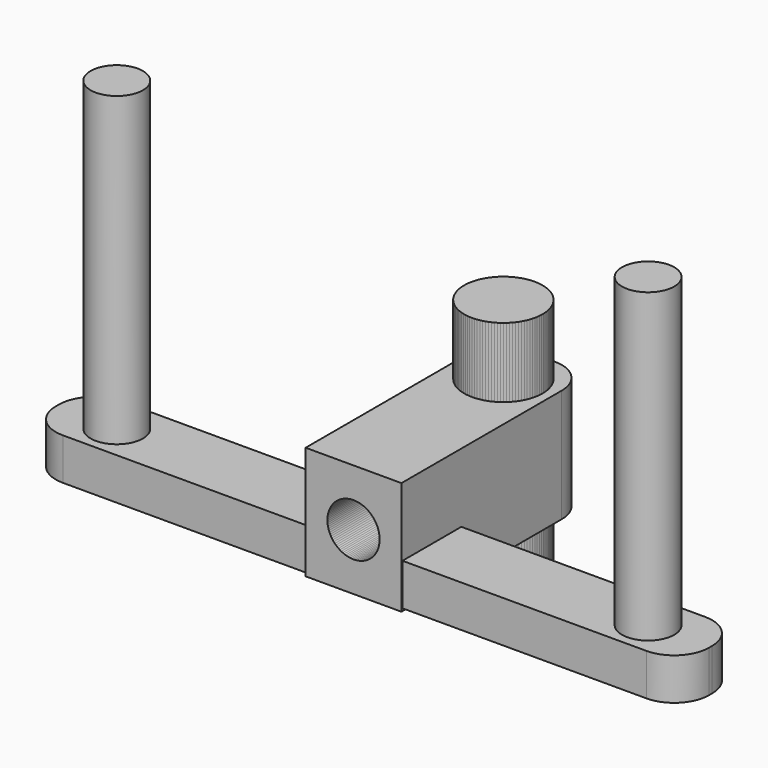
from build123d import *

# Parameters (mm, degrees)
F0_R        = 2.25
F1_DEPTH    = 4
F2_W        = 5.5
F2_H        = 5.5
F3_DEPTH    = 6.5
F4_R        = 2.25
F5_DEPTH    = 4
F6_DEPTH    = 8
F7_R        = 1.5
F8_DEPTH    = 13.5
F9_T1_DEPTH = 16.5
F11_W       = 4.2225685902
F11_H       = 2.4003293365
F12_DEPTH   = 16
F13_R       = 2
F14_R       = 1.5
F15_DEPTH   = 20


# Not quite as in the source:
# - a fillet or chamfer that OpenCascade refuses, or shapes differently, is made with other operations: its cross-section is extruded or revolved along the edge and cut away or added


with BuildPart() as f1:
    # F0 (on Top) → F1 (new body)
    with BuildSketch(Plane.XY):
        Circle(F0_R)
    extrude(amount=F1_DEPTH)

    # F2 (on face) → F3 (join)
    with BuildSketch(Plane.XY.offset(4)):
        Rectangle(F2_W, F2_H)
    extrude(amount=F3_DEPTH)

    # F4 (on face) → F5 (join)
    with BuildSketch(Plane.XY.offset(10.5)):
        Circle(F4_R)
    extrude(amount=F5_DEPTH)

    # F6 (add): a face of the model
    f6_faces = [f1.faces().sort_by_distance(p)[0] for p in [
        (0, -2.75, 7.25),
    ]]
    extrude(f6_faces, amount=F6_DEPTH)

    # F7 (on face) → F8 (cut, through all)
    with BuildSketch(Plane.XZ.offset(10.75)):
        with Locations((0, 7.25)):
            Circle(F7_R)
    extrude(amount=-F8_DEPTH, mode=Mode.SUBTRACT)

    # F9: fillet of radius 2 on 2 edges, made by hand

    # F9_s2 → F9_t1 (cut)
    with BuildSketch(Plane.XY.offset(-1)):
        with BuildLine():
            ThreePointArc((-0.75, 2.75), (-2.1642135624, 2.1642135624), (-2.75, 0.75))
            Line((-2.75, 0.75), (-2.75, 2.75))
            Line((-2.75, 2.75), (-0.75, 2.75))
        make_face()
        with BuildLine():
            ThreePointArc((0.75, 2.75), (2.1642135624, 2.1642135624), (2.75, 0.75))
            Line((2.75, 0.75), (2.75, 2.75))
            Line((2.75, 2.75), (0.75, 2.75))
        make_face()
    extrude(amount=F9_T1_DEPTH, mode=Mode.SUBTRACT)

    # F11 (on face) → F12 (join)
    with BuildSketch(Plane.YZ.offset(2.75)):
        with Locations((-8.5641460028, 5.3448951803)):
            Rectangle(F11_W, F11_H)
    extrude(amount=F12_DEPTH)

    # F13
    f13_edges = [f1.edges().sort_by_distance(p)[0] for p in [
        (18.75, -10.67543, 5.344895),
        (18.75, -6.452862, 5.344895),
    ]]
    fillet(f13_edges, radius=F13_R)

    # F14 (on face) → F15 (join)
    with BuildSketch(Plane(origin=(0, 0, 4.1447305121), x_dir=(1, 0, 0), z_dir=(0, 0, -1))):
        with Locations((15.25, 8.6754302979)):
            Circle(F14_R)
    extrude(amount=-F15_DEPTH)


with BuildPart() as f16_1:
    # F16: instance of F1
    add(f1.part.mirror(Plane.YZ))


solid = Compound([f1.part, f16_1.part])
